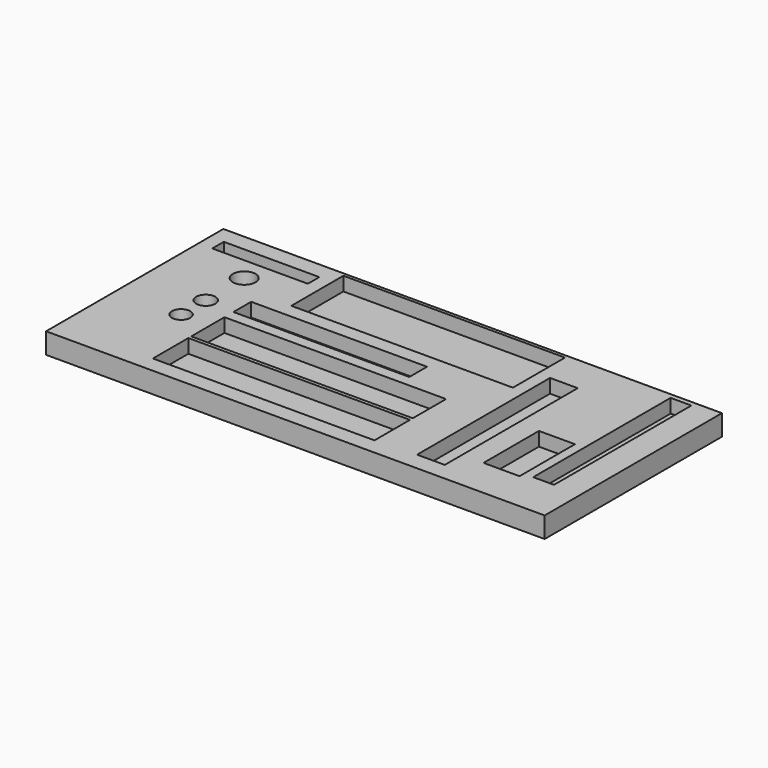
from build123d import *

# Parameters (mm, degrees)
F0_W      = 457.2
F0_H      = 203.2
F1_DEPTH  = 19.05
F2_W      = 203.2
F2_H      = 59.69
F3_R      = 10.414
F3_R_2    = 8.763
F3_R_3    = 8.382
F5_DEPTH  = 19.05
F6_W      = 87.63
F6_H      = 13.208
F11_DEPTH = 12.7
F8_W      = 161.29
F8_H      = 20.32
F8_W_2    = 203.2
F8_H_2    = 38.1
F8_H_3    = 40.64
F12_DEPTH = 12.7
F9_W      = 25.4
F9_H      = 152.4
F10_W     = 33.02
F10_H     = 63.5
F13_DEPTH = 12.7
F7_W      = 19.05
F7_H      = 157.48
F14_DEPTH = 12.7
F15_DEPTH = 12.7
F16_DEPTH = 12.7


# Not quite as in the source:
# - the program builds the solid bodies; features that only make, move or delete a surface that nothing else refers to are left out


with BuildPart() as f1:
    # F0 (on Top) → F1 (new body)
    with BuildSketch(Plane.XY):
        with Locations((-168.2645873785, 42.8677027285)):
            Rectangle(F0_W, F0_H)
    extrude(amount=F1_DEPTH)

    # F2 (on face) + F3 (on face) → F5 (join)
    with BuildSketch(Plane.XY.offset(19.05)):
        with Locations((-182.8039201736, 111.6589910698)):
            Rectangle(F2_W, F2_H)
    with BuildSketch(Plane.XY.offset(19.05)):
        with Locations((-337.6098275185, 94.2841172218)):
            Circle(F3_R)
        with Locations((-337.6098275185, 50.222992897)):
            Circle(F3_R_2)
        with Locations((-337.6098275185, 21.9573695213)):
            Circle(F3_R_3)
    extrude(amount=-F5_DEPTH)

    # F6 (on face) → F11 (cut)
    with BuildSketch(Plane.XY.offset(19.05)):
        with Locations((-340.3499591923, 122.5030114927)):
            Rectangle(F6_W, F6_H)
    extrude(amount=-F11_DEPTH, mode=Mode.SUBTRACT)

    # F8 (on face) → F12 (cut)
    with BuildSketch(Plane.XY.offset(19.05)):
        with Locations((-230.1238527489, 58.5634791589)):
            Rectangle(F8_W, F8_H)
        with Locations((-209.1688527489, 19.05)):
            Rectangle(F8_W_2, F8_H_2)
        with Locations((-209.1688527489, -23.6032848585)):
            Rectangle(F8_W_2, F8_H_3)
    extrude(amount=-F12_DEPTH, mode=Mode.SUBTRACT)

    # F9 (on face) + F10 (on face) → F13 (cut)
    with BuildSketch(Plane.XY.offset(19.05)):
        with Locations((-57.1830842316, 34.0140676022)):
            Rectangle(F9_W, F9_H)
    with BuildSketch(Plane.XY.offset(19.05)):
        with Locations((-8.2516423559, 9.3228359818)):
            Rectangle(F10_W, F10_H)
    extrude(amount=-F13_DEPTH, mode=Mode.SUBTRACT)

    # F7 (on face) → F14 (cut)
    with BuildSketch(Plane.XY.offset(19.05)):
        with Locations((26.3747599661, 61.2730749154)):
            Rectangle(F7_W, F7_H)
    extrude(amount=-F14_DEPTH, mode=Mode.SUBTRACT)

    # F2 (on face) → F15 (cut)
    with BuildSketch(Plane.XY.offset(19.05)):
        with Locations((-182.8039201736, 111.6589910698)):
            Rectangle(F2_W, F2_H)
    extrude(amount=-F15_DEPTH, mode=Mode.SUBTRACT)

    # F3 (on face) → F16 (cut)
    with BuildSketch(Plane.XY.offset(19.05)):
        with Locations((-337.6098275185, 94.2841172218)):
            Circle(F3_R)
        with Locations((-337.6098275185, 50.222992897)):
            Circle(F3_R_2)
        with Locations((-337.6098275185, 21.9573695213)):
            Circle(F3_R_3)
    extrude(amount=-F16_DEPTH, mode=Mode.SUBTRACT)


solid = f1.part
